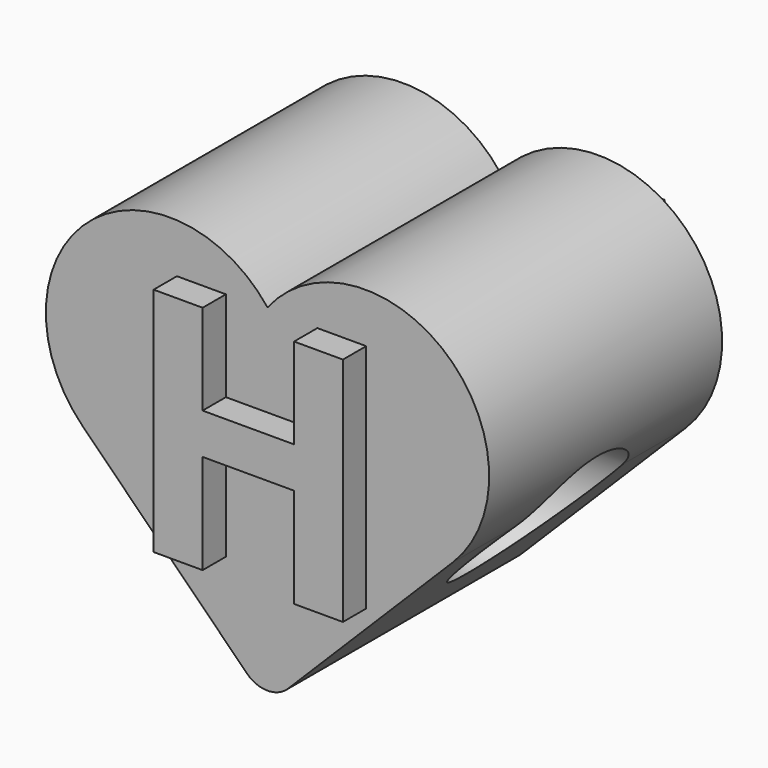
from build123d import *

# Parameters (mm, degrees)
F1_DEPTH     = 10
F2_TEXT_SIZE = 11.1111111111
F3_DEPTH     = 1
F5_R         = 2.5
F6_DEPTH     = 12.5
F7_R         = 1
F8_TEXT_SIZE = 9.7222222222
F9_DEPTH     = 1


# Not quite as in the source:
# - Text() gives the source's letters only with a copy of the font that has no kerning and outlines rounded to 1/6400 em; it was checked with that copy


with BuildPart() as f1:
    # F0 (on Front) → F1 (new body)
    with BuildSketch(Plane.XZ):
        with BuildLine():
            Line((-6.3639610307, 1.3728261765), (0, -4.9911348542))
            Line((0, -4.9911348542), (0, 7.0088651458))
            ThreePointArc((0, 7.0088651458), (-6.1761214571, 7.5716945831), (-6.3639610307, 1.3728261765))
        make_face()
        with BuildLine():
            Line((0, 7.0088651458), (0, -4.9911348542))
            Line((0, -4.9911348542), (6.3639610307, 1.3728261765))
            ThreePointArc((6.3639610307, 1.3728261765), (6.1761214571, 7.5716945831), (0, 7.0088651458))
        make_face()
    extrude(amount=F1_DEPTH)

    # F2 (on face) → F3 (join)
    with BuildSketch(Plane.XZ.offset(10)):
        with Locations((-4.109375, -0.9911348542)):
            Text('H', F2_TEXT_SIZE, font='Open Sans', font_style=FontStyle.BOLD, text_align=(TextAlign.LEFT, TextAlign.BOTTOM))
    extrude(amount=F3_DEPTH)

    # F5 (on Right) → F6 (cut, symmetric)
    with BuildSketch(Plane.YZ):
        with Locations((-5, 0.3728261765)):
            Circle(F5_R)
    extrude(amount=F6_DEPTH, both=True, mode=Mode.SUBTRACT)

    # F7
    f7_edges = [f1.edges().sort_by_distance(p)[0] for p in [
        (0, -5, -4.991135),
    ]]
    fillet(f7_edges, radius=F7_R)

    # F8 (on face) → F9 (join)
    with BuildSketch(Plane(origin=(0, 0, 0), x_dir=(-1, 0, 0), z_dir=(0, 1, 0))):
        with Locations((-5.7102864583, 0.4230787081)):
            Text('56', F8_TEXT_SIZE, font='Open Sans', font_style=FontStyle.BOLD, text_align=(TextAlign.LEFT, TextAlign.BOTTOM))
    extrude(amount=F9_DEPTH)


solid = f1.part
